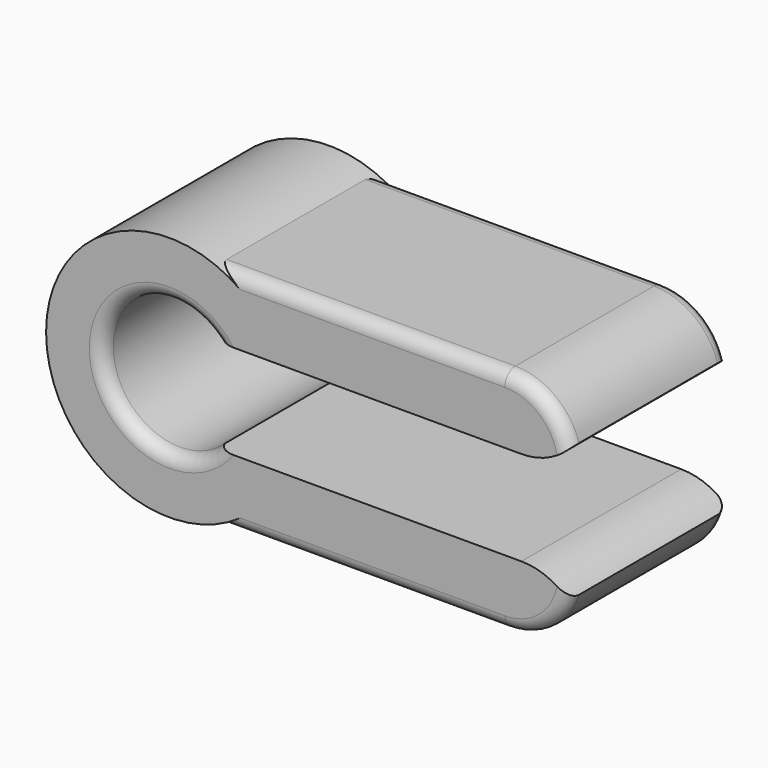
from build123d import *

# Parameters (mm, degrees)
F1_DEPTH    = 15
F2_T1_DEPTH = 56.5812984693
F3_R        = 1


# Not quite as in the source:
# - a fillet or chamfer that OpenCascade refuses, or shapes differently, is made with other operations: its cross-section is extruded or revolved along the edge and cut away or added


with BuildPart() as f1:
    # F0 (on Front) → F1 (new body)
    with BuildSketch(Plane.XZ):
        with BuildLine():
            Line((30.5210083783, 8.55), (0.5210083783, 8.55))
            ThreePointArc((0.5210083783, 8.55), (-12.2466210045, 0), (0.5210083783, -8.55))
            Line((0.5210083783, -8.55), (30.5210083783, -8.55))
            Line((30.5210083783, -8.55), (26.9854744724, -5.0144660941))
            ThreePointArc((26.9854744724, -5.0144660941), (25.3633577283, -3.9306023374), (23.4499405664, -3.55))
            Line((23.4499405664, -3.55), (0.5210083783, -3.55))
            ThreePointArc((0.5210083783, -3.55), (-8, 0), (0.5210083783, 3.55))
            Line((0.5210083783, 3.55), (23.4499405664, 3.55))
            ThreePointArc((23.4499405664, 3.55), (25.3633577283, 3.9306023374), (26.9854744724, 5.0144660941))
            Line((26.9854744724, 5.0144660941), (30.5210083783, 8.55))
        make_face()
    extrude(amount=F1_DEPTH)

    # F2: fillet of radius 5 on 2 edges, made by hand

    # F2_s2 → F2_t1 (cut)
    with BuildSketch(Plane.XZ.offset(-20.7906492346)):
        with BuildLine():
            ThreePointArc((22.2047486844, -8.55), (25.1777664719, -7.5700951774), (26.9854744724, -5.0144660941))
            Line((26.9854744724, -5.0144660941), (30.5210083783, -8.55))
            Line((30.5210083783, -8.55), (22.2047486844, -8.55))
        make_face()
        with BuildLine():
            ThreePointArc((26.9854744724, 5.0144660941), (25.1777664719, 7.5700951774), (22.2047486844, 8.55))
            Line((22.2047486844, 8.55), (30.5210083783, 8.55))
            Line((30.5210083783, 8.55), (26.9854744724, 5.0144660941))
        make_face()
    extrude(amount=F2_T1_DEPTH, mode=Mode.SUBTRACT)

    # F3
    f3_edges = [f1.edges().sort_by_distance(p)[0] for p in [
        (11.362879, 0, -8.55),
        (11.362879, -15, -8.55),
        (11.362879, -15, 8.55),
        (11.362879, 0, 8.55),
        (-8, -15, 0),
        (-8, 0, 0),
        (25.177766, 0, 7.570095),
        (25.177766, -15, 7.570095),
        (25.177766, 0, -7.570095),
        (25.177766, -15, -7.570095),
    ]]
    fillet(f3_edges, radius=F3_R)


solid = f1.part
